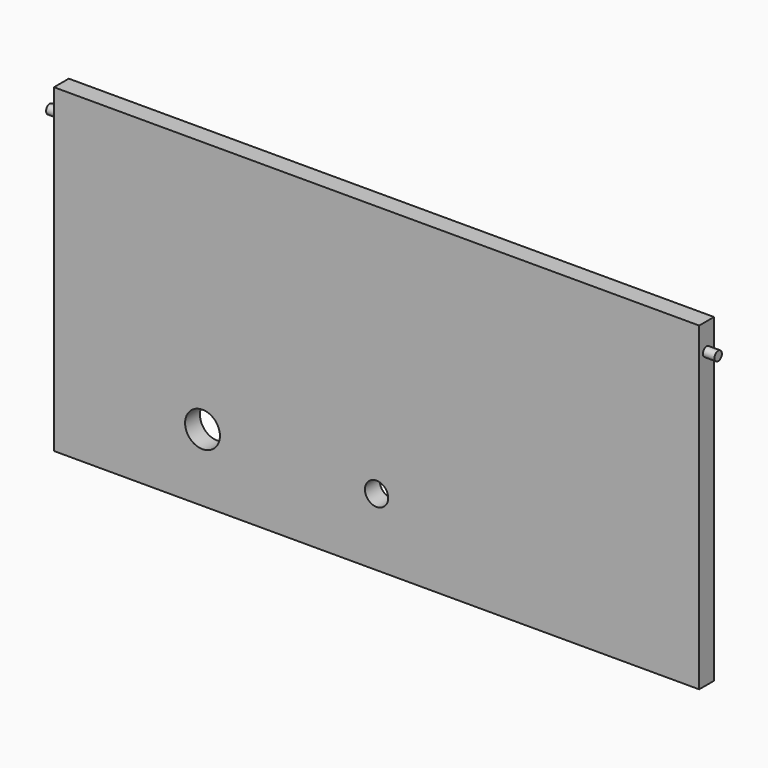
from build123d import *

# Parameters (mm, degrees)
F0_W     = 278
F0_H     = 138
F0_R     = 7.5
F0_R_2   = 5
F1_DEPTH = 8
F2_R     = 2
F3_DEPTH = 5


with BuildPart() as f1:
    # F0 (on Front) → F1 (new body)
    with BuildSketch(Plane.XZ):
        Rectangle(F0_W, F0_H)
        with Locations((-75, -40)):
            Circle(F0_R, mode=Mode.SUBTRACT)
        with Locations((0, -40)):
            Circle(F0_R_2, mode=Mode.SUBTRACT)
    extrude(amount=F1_DEPTH)



with BuildPart() as f3:
    # F2 (on face) → F3 (new body)
    with BuildSketch(Plane.YZ.offset(139)):
        with Locations((-4, 57.5)):
            Circle(F2_R)
    extrude(amount=F3_DEPTH)


with BuildPart() as f1_1:
    add(f1.part)

    add(f3.part)  # F4 merges F3
    # F4: F3 across plane
    add(f3.part.mirror(Plane.YZ))


solid = f1_1.part
